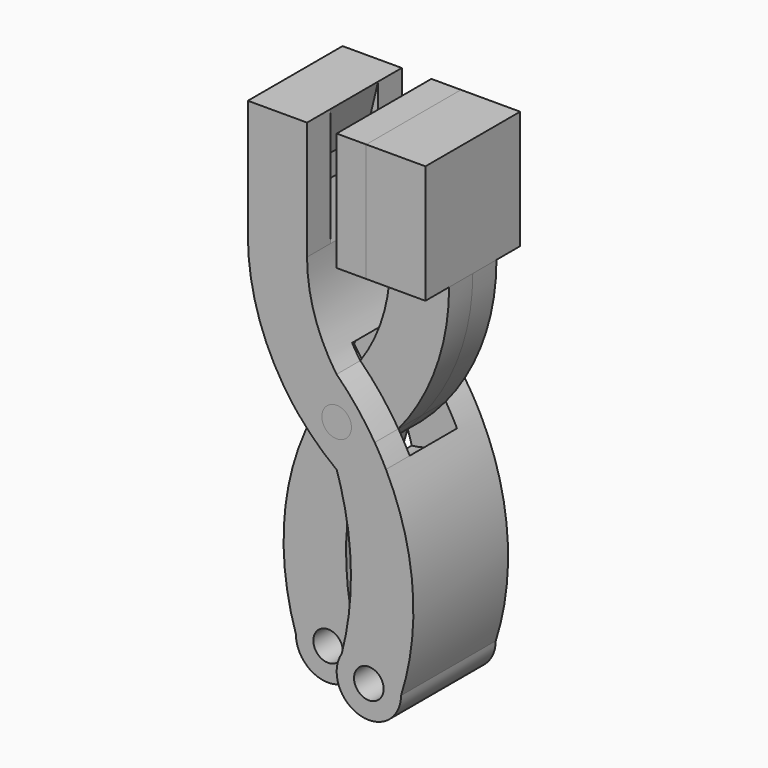
from build123d import *

# Parameters (mm, degrees)
F1_DEPTH      = 12.7
F1_DEPTH_BACK = 12.7
F2_DEPTH      = 6.35
F2_DEPTH_BACK = 6.35
F3_DEPTH      = 6.35
F3_DEPTH_BACK = 6.35
F0_W          = 6.35
F0_H          = 25.4
F4_DEPTH      = 12.7
F4_DEPTH_BACK = 12.7
F0_R          = 3.175
F5_DEPTH      = 6.35
F5_DEPTH_BACK = 6.35
F6_DEPTH      = 12.7
F6_DEPTH_BACK = 12.7
F7_DEPTH      = 6.35
F7_DEPTH_BACK = 6.35
F8_DEPTH      = 12.7
F8_DEPTH_BACK = 12.7


with BuildPart() as f1:
    # F0 (on Front) → F1 (new body, two sides)
    with BuildSketch(Plane.XZ) as f1_sk:
        Polygon((-8.827155169, -10.3124072454), (-6.35, 0), (-19.05, 0), (-19.05, -25.4), (-6.35, -25.4), (-8.827155169, -15.0875927546), (-12.9381986335, -19.05), (-12.9381986335, -12.7), (-12.9381986335, -6.35), align=None)
        Polygon((-6.35, -25.4), (-6.35, 0), (-8.827155169, -10.3124072454), (-12.9381986335, -6.35), (-12.9381986335, -12.7), (-12.9381986335, -19.05), (-8.827155169, -15.0875927546), align=None)
    extrude(amount=-F1_DEPTH)
    extrude(f1_sk.sketch, amount=F1_DEPTH_BACK)


with BuildPart() as f1b:
    # F0 (on Front) → F1, piece 2 (new body, two sides)
    with BuildSketch(Plane.XZ) as f1_2_sk:
        Polygon((19.05, 0), (6.35, 0), (8.827155169, -10.3124072454), (12.9381986335, -6.35), (12.9381986335, -12.7), (12.9381986335, -19.05), (8.827155169, -15.0875927546), (6.35, -25.4), (19.05, -25.4), align=None)
        Polygon((8.827155169, -10.3124072454), (6.35, 0), (6.35, -25.4), (8.827155169, -15.0875927546), (12.9381986335, -19.05), (12.9381986335, -12.7), (12.9381986335, -6.35), align=None)
    extrude(amount=-F1_DEPTH)
    extrude(f1_2_sk.sketch, amount=F1_DEPTH_BACK)


with BuildPart() as f2_tool:
    # F0 (on Front) → F2 (new body, two sides)
    with BuildSketch(Plane.XZ) as f2_sk:
        Polygon((8.827155169, -10.3124072454), (6.35, 0), (6.35, -25.4), (8.827155169, -15.0875927546), (12.9381986335, -19.05), (12.9381986335, -12.7), (12.9381986335, -6.35), align=None)
        Polygon((-6.35, -25.4), (-6.35, 0), (-8.827155169, -10.3124072454), (-12.9381986335, -6.35), (-12.9381986335, -12.7), (-12.9381986335, -19.05), (-8.827155169, -15.0875927546), align=None)
    extrude(amount=F2_DEPTH)
    extrude(f2_sk.sketch, amount=-F2_DEPTH_BACK)


with BuildPart() as f1_1:
    add(f1.part)

    # F2: cut by f2_tool
    add(f2_tool.part, mode=Mode.SUBTRACT)

    # F0 (on Front) → F6 (join, two sides)
    with BuildSketch(Plane.XZ) as f6_sk:
        with BuildLine():
            ThreePointArc((-1.7703138016, -42.6892323508), (-5.1856702357, -34.3427495905), (-6.35, -25.4))
            Line((-6.35, -25.4), (-19.05, -25.4))
            ThreePointArc((-19.05, -25.4), (-17.1147005889, -38.8384480167), (-11.4660888148, -51.1847208929))
            ThreePointArc((-11.4660888148, -51.1847208929), (-7.8640905354, -45.515061734), (-1.7703138016, -42.6892323508))
        make_face()
        with BuildLine():
            ThreePointArc((-8.1699275215, -55.6977049698), (-4.3890156004, -50.3459576296), (0, -45.4804631421))
            ThreePointArc((0, -45.4804631421), (-0.9181956043, -44.1058022562), (-1.7703138016, -42.6892323508))
            ThreePointArc((-1.7703138016, -42.6892323508), (-7.8640905354, -45.515061734), (-11.4660888148, -51.1847208929))
            ThreePointArc((-11.4660888148, -51.1847208929), (-9.8842619862, -53.4896029249), (-8.1699275215, -55.6977049698))
        make_face()
        with BuildLine():
            Line((0, -51.315231571), (0, -45.4804631421))
            ThreePointArc((0, -45.4804631421), (-4.3890156004, -50.3459576296), (-8.1699275215, -55.6977049698))
            ThreePointArc((-8.1699275215, -55.6977049698), (-4.3171295265, -59.8419575549), (0, -63.5))
            Line((0, -63.5), (0, -57.665231571))
            ThreePointArc((0, -57.665231571), (-3.175, -54.490231571), (0, -51.315231571))
        make_face()
        with BuildLine():
            ThreePointArc((8.1699275215, -55.6977049698), (4.3890156004, -50.3459576296), (0, -45.4804631421))
            Line((0, -45.4804631421), (0, -51.315231571))
            ThreePointArc((0, -51.315231571), (2.2450640303, -52.2451675408), (3.175, -54.490231571))
            ThreePointArc((3.175, -54.490231571), (2.2450640303, -56.7352956013), (0, -57.665231571))
            Line((0, -57.665231571), (0, -63.5))
            ThreePointArc((0, -63.5), (4.3171295265, -59.8419575549), (8.1699275215, -55.6977049698))
        make_face()
        with BuildLine():
            ThreePointArc((13.816319406, -101.6703248024), (16.2998142634, -80.5187022847), (10.5831374671, -60.0033790301))
            ThreePointArc((10.5831374671, -60.0033790301), (6.5593543364, -64.4588054029), (0.8753606705, -66.3911280603))
            ThreePointArc((0.8753606705, -66.3911280603), (3.0617092136, -82.1370373381), (1.0895635546, -97.9112067437))
            ThreePointArc((1.0895635546, -97.9112067437), (0.282876498, -99.6782440765), (0, -101.6))
            ThreePointArc((0, -101.6), (8.94874e-05, -101.6351624012), (0, -101.6703248024))
            ThreePointArc((0, -101.6703248024), (6.908159703, -108.5434115916), (13.816319406, -101.6703248024))
        make_face()
        with Locations((6.908159703, -101.6351624012)):
            Circle(F0_R, mode=Mode.SUBTRACT)
        with BuildLine():
            ThreePointArc((10.5831374671, -60.0033790301), (9.424729686, -57.8235288213), (8.1699275215, -55.6977049698))
            ThreePointArc((8.1699275215, -55.6977049698), (4.3171295265, -59.8419575549), (0, -63.5))
            ThreePointArc((0, -63.5), (0.4556473184, -64.9401240807), (0.8753606705, -66.3911280603))
            ThreePointArc((0.8753606705, -66.3911280603), (6.5593543364, -64.4588054029), (10.5831374671, -60.0033790301))
        make_face()
        with BuildLine():
            ThreePointArc((13.816319406, -101.6703248024), (16.2998142634, -80.5187022847), (10.5831374671, -60.0033790301))
            ThreePointArc((10.5831374671, -60.0033790301), (6.5593543364, -64.4588054029), (0.8753606705, -66.3911280603))
            ThreePointArc((0.8753606705, -66.3911280603), (3.0617092136, -82.1370373381), (1.0895635546, -97.9112067437))
            ThreePointArc((1.0895635546, -97.9112067437), (0.282876498, -99.6782440765), (0, -101.6))
            ThreePointArc((0, -101.6), (8.94874e-05, -101.6351624012), (0, -101.6703248024))
            ThreePointArc((0, -101.6703248024), (6.908159703, -108.5434115916), (13.816319406, -101.6703248024))
        make_face()
        with Locations((6.908159703, -101.6351624012)):
            Circle(F0_R, mode=Mode.SUBTRACT)
    extrude(amount=F6_DEPTH)
    extrude(f6_sk.sketch, amount=-F6_DEPTH_BACK)

    # F0 (on Front) → F7 (cut, two sides)
    with BuildSketch(Plane.XZ) as f7_sk:
        with BuildLine():
            ThreePointArc((-8.1699275215, -55.6977049698), (-4.3890156004, -50.3459576296), (0, -45.4804631421))
            ThreePointArc((0, -45.4804631421), (-0.9181956043, -44.1058022562), (-1.7703138016, -42.6892323508))
            ThreePointArc((-1.7703138016, -42.6892323508), (-7.8640905354, -45.515061734), (-11.4660888148, -51.1847208929))
            ThreePointArc((-11.4660888148, -51.1847208929), (-9.8842619862, -53.4896029249), (-8.1699275215, -55.6977049698))
        make_face()
        with BuildLine():
            Line((0, -51.315231571), (0, -45.4804631421))
            ThreePointArc((0, -45.4804631421), (-4.3890156004, -50.3459576296), (-8.1699275215, -55.6977049698))
            ThreePointArc((-8.1699275215, -55.6977049698), (-4.3171295265, -59.8419575549), (0, -63.5))
            Line((0, -63.5), (0, -57.665231571))
            ThreePointArc((0, -57.665231571), (-3.175, -54.490231571), (0, -51.315231571))
        make_face()
        with BuildLine():
            ThreePointArc((8.1699275215, -55.6977049698), (4.3890156004, -50.3459576296), (0, -45.4804631421))
            Line((0, -45.4804631421), (0, -51.315231571))
            ThreePointArc((0, -51.315231571), (2.2450640303, -52.2451675408), (3.175, -54.490231571))
            ThreePointArc((3.175, -54.490231571), (2.2450640303, -56.7352956013), (0, -57.665231571))
            Line((0, -57.665231571), (0, -63.5))
            ThreePointArc((0, -63.5), (4.3171295265, -59.8419575549), (8.1699275215, -55.6977049698))
        make_face()
        with BuildLine():
            ThreePointArc((10.5831374671, -60.0033790301), (9.424729686, -57.8235288213), (8.1699275215, -55.6977049698))
            ThreePointArc((8.1699275215, -55.6977049698), (4.3171295265, -59.8419575549), (0, -63.5))
            ThreePointArc((0, -63.5), (0.4556473184, -64.9401240807), (0.8753606705, -66.3911280603))
            ThreePointArc((0.8753606705, -66.3911280603), (6.5593543364, -64.4588054029), (10.5831374671, -60.0033790301))
        make_face()
    extrude(amount=F7_DEPTH, mode=Mode.SUBTRACT)
    extrude(f7_sk.sketch, amount=-F7_DEPTH_BACK, mode=Mode.SUBTRACT)


with BuildPart() as f1b_1:
    add(f1b.part)

    # F2: cut by f2_tool
    add(f2_tool.part, mode=Mode.SUBTRACT)

    # F0 (on Front) → F5 (join, two sides)
    with BuildSketch(Plane.XZ) as f5_sk:
        with BuildLine():
            Line((19.05, -25.4), (6.35, -25.4))
            ThreePointArc((6.35, -25.4), (4.7246809294, -35.9302837094), (0, -45.4804631421))
            ThreePointArc((0, -45.4804631421), (4.3890156004, -50.3459576296), (8.1699275215, -55.6977049698))
            ThreePointArc((8.1699275215, -55.6977049698), (16.2475266926, -41.4960158391), (19.05, -25.4))
        make_face()
        with BuildLine():
            ThreePointArc((8.1699275215, -55.6977049698), (4.3890156004, -50.3459576296), (0, -45.4804631421))
            Line((0, -45.4804631421), (0, -51.315231571))
            ThreePointArc((0, -51.315231571), (2.2450640303, -52.2451675408), (3.175, -54.490231571))
            ThreePointArc((3.175, -54.490231571), (2.2450640303, -56.7352956013), (0, -57.665231571))
            Line((0, -57.665231571), (0, -63.5))
            ThreePointArc((0, -63.5), (4.3171295265, -59.8419575549), (8.1699275215, -55.6977049698))
        make_face()
        with BuildLine():
            Line((0, -51.315231571), (0, -45.4804631421))
            ThreePointArc((0, -45.4804631421), (-4.3890156004, -50.3459576296), (-8.1699275215, -55.6977049698))
            ThreePointArc((-8.1699275215, -55.6977049698), (-4.3171295265, -59.8419575549), (0, -63.5))
            Line((0, -63.5), (0, -57.665231571))
            ThreePointArc((0, -57.665231571), (-3.175, -54.490231571), (0, -51.315231571))
        make_face()
        with BuildLine():
            ThreePointArc((0, -63.5), (-4.3171295265, -59.8419575549), (-8.1699275215, -55.6977049698))
            ThreePointArc((-8.1699275215, -55.6977049698), (-16.0538027814, -78.0624584307), (-13.816319406, -101.6703248024))
            ThreePointArc((-13.816319406, -101.6703248024), (-6.908159703, -108.5434115916), (0, -101.6703248024))
            ThreePointArc((0, -101.6703248024), (-8.94874e-05, -101.6351624012), (0, -101.6))
            ThreePointArc((0, -101.6), (-0.282876498, -99.6782440765), (-1.0895635546, -97.9112067437))
            ThreePointArc((-1.0895635546, -97.9112067437), (-3.0326733006, -80.626829153), (0, -63.5))
        make_face()
        with Locations((-6.908159703, -101.6351624012)):
            Circle(F0_R, mode=Mode.SUBTRACT)
    extrude(amount=F5_DEPTH)
    extrude(f5_sk.sketch, amount=-F5_DEPTH_BACK)


with BuildPart() as f3:
    # F0 (on Front) → F3 (new body, two sides)
    with BuildSketch(Plane.XZ) as f3_sk:
        Polygon((8.827155169, -10.3124072454), (6.35, 0), (6.35, -25.4), (8.827155169, -15.0875927546), (12.9381986335, -19.05), (12.9381986335, -12.7), (12.9381986335, -6.35), align=None)
    extrude(amount=F3_DEPTH)
    extrude(f3_sk.sketch, amount=-F3_DEPTH_BACK)

    # F0 (on Front) → F4 (join, two sides)
    with BuildSketch(Plane.XZ) as f4_sk:
        with Locations((3.175, -12.7)):
            Rectangle(F0_W, F0_H)
    extrude(amount=F4_DEPTH)
    extrude(f4_sk.sketch, amount=-F4_DEPTH_BACK)


with BuildPart() as f8:
    # F0 (on Front) → F8 (new body, two sides)
    with BuildSketch(Plane.XZ) as f8_sk:
        with BuildLine():
            Line((0, -57.665231571), (0, -51.315231571))
            ThreePointArc((0, -51.315231571), (-3.175, -54.490231571), (0, -57.665231571))
        make_face()
        with BuildLine():
            ThreePointArc((3.175, -54.490231571), (2.2450640303, -52.2451675408), (0, -51.315231571))
            Line((0, -51.315231571), (0, -57.665231571))
            ThreePointArc((0, -57.665231571), (2.2450640303, -56.7352956013), (3.175, -54.490231571))
        make_face()
    extrude(amount=F8_DEPTH)
    extrude(f8_sk.sketch, amount=-F8_DEPTH_BACK)


solid = Compound([f1_1.part, f1b_1.part, f3.part, f8.part])
